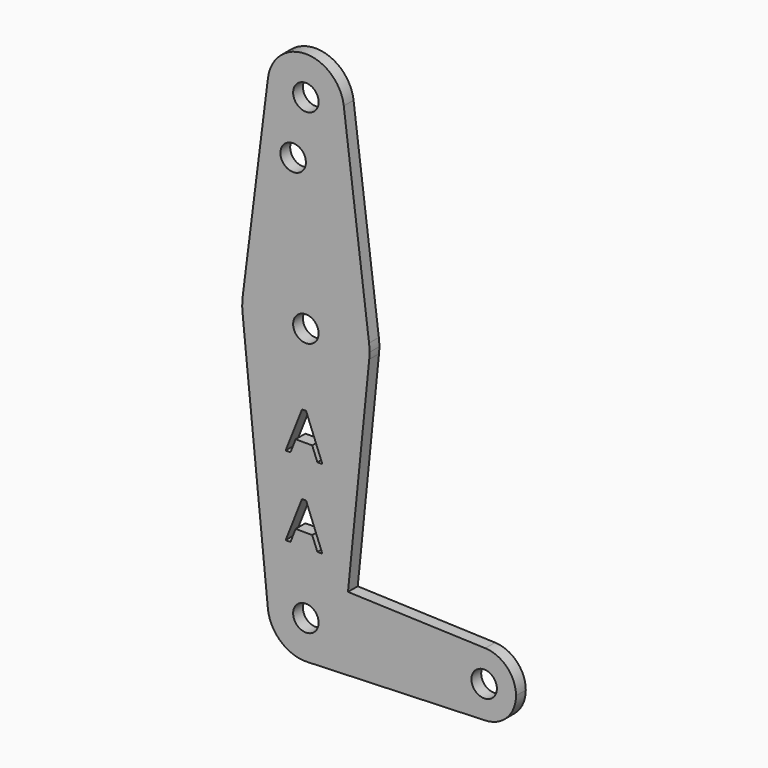
from build123d import *

# Parameters (mm, degrees)
F0_R     = 3.175
F1_DEPTH = 3.048


with BuildPart() as f1:
    # F0 (on Front) → F1 (new body)
    with BuildSketch(Plane.XZ):
        with BuildLine():
            ThreePointArc((9.4772553384, -0.9525), (9.5130563464, -0.4768479324), (9.525, 0))
            ThreePointArc((9.525, 0), (6.8544082857, 6.6138273378), (0.3401785714, 9.5189234444))
            ThreePointArc((0.3401785714, 9.5189234444), (-6.948684782, 6.5147068085), (-9.4772553384, -0.9525))
            ThreePointArc((-9.4772553384, -0.9525), (-6.2623833552, -7.1769199322), (0.3401786416, -9.5189234418))
            ThreePointArc((0.3401786416, -9.5189234418), (6.5147068341, -6.948684758), (9.4772553384, -0.9525))
        make_face()
        Circle(F0_R, mode=Mode.SUBTRACT)
        with BuildLine():
            ThreePointArc((0.3401785714, 9.5189234444), (6.8544082857, 6.6138273378), (9.525, 0))
            ThreePointArc((9.525, 0), (9.5130563464, -0.4768479324), (9.4772553384, -0.9525))
            Line((9.4772553384, -0.9525), (10.4932062399, 9.1560838367))
            Line((10.4932062399, 9.1560838367), (0.3401785714, 9.5189234444))
        make_face()
        with BuildLine():
            ThreePointArc((-9.4772553384, -0.9525), (-6.948684782, 6.5147068085), (0.3401785714, 9.5189234444))
            Line((0.3401785714, 9.5189234444), (10.4932062399, 9.1560838367))
            Line((10.4932062399, 9.1560838367), (15.7954255641, 61.9125))
            ThreePointArc((15.7954255641, 61.9125), (0, 47.625), (-15.7954255641, 61.9125))
            Line((-15.7954255641, 61.9125), (-9.4772553384, -0.9525))
        make_face()
        Polygon((4.1081828244, 15.4546830389), (2.8649913232, 15.4546830389), (1.5788532065, 18.7389689503), (-2.5598443184, 18.7389689503), (-3.8301599978, 15.4546830389), (-5.0462273207, 15.4546830389), (-0.9640385005, 25.825160507), (0.0463371378, 25.825160507), align=None, mode=Mode.SUBTRACT)
        Polygon((4.1081828244, 35.1287536323), (2.8649913232, 35.1287536323), (1.5788532065, 38.4130395436), (-2.5598443184, 38.4130395436), (-3.8301599978, 35.1287536323), (-5.0462273207, 35.1287536323), (-0.9640385005, 45.4992311004), (0.0463371378, 45.4992311004), align=None, mode=Mode.SUBTRACT)
        with BuildLine():
            Line((10.4932062399, 9.1560838367), (9.4772553384, -0.9525))
            ThreePointArc((9.4772553384, -0.9525), (6.5147068341, -6.948684758), (0.3401786416, -9.5189234418))
            Line((0.3401786416, -9.5189234418), (44.7334821429, -7.9324362036))
            ThreePointArc((44.7334821429, -7.9324362036), (36.5125, 0), (44.7334821429, 7.9324362036))
            Line((44.7334821429, 7.9324362036), (10.4932062399, 9.1560838367))
        make_face()
        with BuildLine():
            ThreePointArc((-15.7504882737, 65.484375), (-15.8737438155, 63.6997054867), (-15.7954255641, 61.9125))
            ThreePointArc((-15.7954255641, 61.9125), (0, 47.625), (15.7954255641, 61.9125))
            ThreePointArc((15.7954255641, 61.9125), (15.8550939106, 62.7052534459), (15.875, 63.5))
            ThreePointArc((15.875, 63.5), (15.8438414904, 64.4941387366), (15.7504882737, 65.484375))
            ThreePointArc((15.7504882737, 65.484375), (0, 79.375), (-15.7504882737, 65.484375))
        make_face()
        with Locations((0, 63.5)):
            Circle(F0_R, mode=Mode.SUBTRACT)
        with BuildLine():
            ThreePointArc((52.3875, 0), (50.1620069047, 5.5115227815), (44.7334821429, 7.9324362036))
            ThreePointArc((44.7334821429, 7.9324362036), (36.5125, 0), (44.7334821429, -7.9324362036))
            ThreePointArc((44.7334821429, -7.9324362036), (50.1620069047, -5.5115227815), (52.3875, 0))
        make_face()
        with Locations((44.45, 0)):
            Circle(F0_R, mode=Mode.SUBTRACT)
        with BuildLine():
            Line((-9.4502929642, 115.490625), (-15.7504882737, 65.484375))
            ThreePointArc((-15.7504882737, 65.484375), (0, 79.375), (15.7504882737, 65.484375))
            Line((15.7504882737, 65.484375), (9.4502929642, 115.490625))
            ThreePointArc((9.4502929642, 115.490625), (9.5063048942, 114.896483242), (9.525, 114.3))
            ThreePointArc((9.525, 114.3), (-0.596483242, 104.7936951058), (-9.4502929642, 115.490625))
        make_face()
        with Locations((-3.175, 100.0252)):
            Circle(F0_R, mode=Mode.SUBTRACT)
        with BuildLine():
            ThreePointArc((9.4502929642, 115.490625), (0, 123.825), (-9.4502929642, 115.490625))
            ThreePointArc((-9.4502929642, 115.490625), (-0.596483242, 104.7936951058), (9.525, 114.3))
            ThreePointArc((9.525, 114.3), (9.5063048942, 114.896483242), (9.4502929642, 115.490625))
        make_face()
        with Locations((0, 114.3)):
            Circle(F0_R, mode=Mode.SUBTRACT)
    extrude(amount=F1_DEPTH)


solid = f1.part
